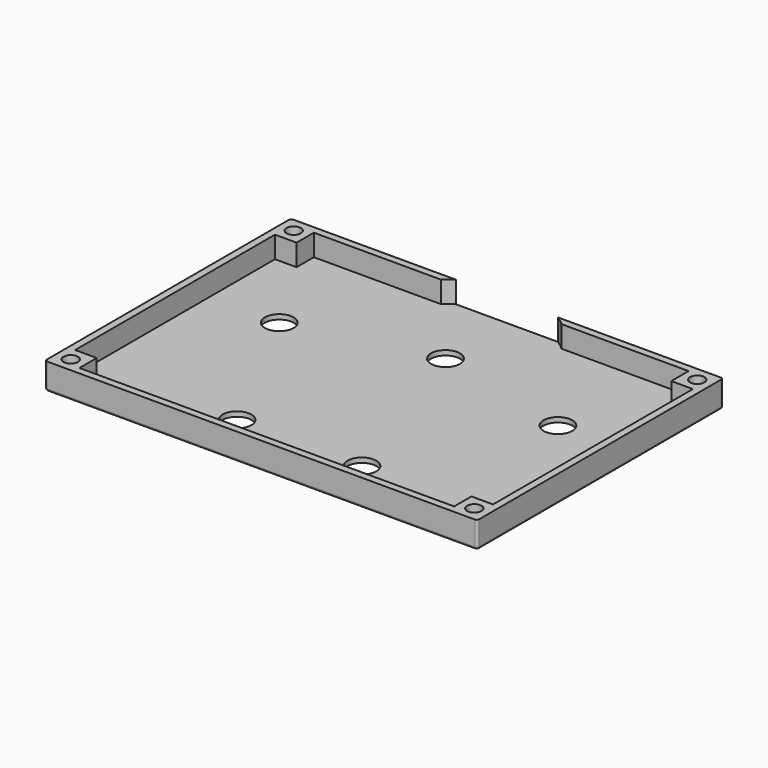
from build123d import *

# Parameters (mm, degrees)
F0_W      = 90
F0_H      = 64
F1_DEPTH  = 1
F3_W      = 90
F3_H      = 64
F3_W_2    = 87
F3_H_2    = 61
F4_DEPTH  = 4.5
F5_R      = 3
F6_DEPTH  = 1.001
F8_DEPTH  = 4.501
F10_W     = 4.5
F10_H     = 4.5
F11_DEPTH = 4.5
F12_R     = 1.5
F13_DEPTH = 5.501
F14_R     = 0.5
F16_SIZE  = 0.2


# Not quite as in the source:
# - two fillets or chamfers of one size are made in one step


with BuildPart() as f1:
    # F0 (on Top) → F1 (new body)
    with BuildSketch(Plane.XY):
        with Locations((45, 32)):
            Rectangle(F0_W, F0_H)
    extrude(amount=F1_DEPTH)

    # F3 (on face) → F4 (join)
    with BuildSketch(Plane.XY.offset(1)):
        with Locations((45, 32)):
            Rectangle(F3_W, F3_H)
        with Locations((45, 32)):
            Rectangle(F3_W_2, F3_H_2, mode=Mode.SUBTRACT)
    extrude(amount=F4_DEPTH)

    # F5 (on face) → F6 (cut, through all)
    with BuildSketch(Plane.XY.offset(1)):
        with Locations((16, 41)):
            Circle(F5_R)
        with Locations((45, 48)):
            Circle(F5_R)
        with Locations((32, 10)):
            Circle(F5_R)
        with Locations((58, 10)):
            Circle(F5_R)
        with Locations((74, 41)):
            Circle(F5_R)
    extrude(amount=-F6_DEPTH, mode=Mode.SUBTRACT)

    # F7 (on face) → F8 (cut, through all)
    with BuildSketch(Plane.XY.offset(1)):
        with BuildLine():
            ThreePointArc((34.3868006709, 64), (35.920722141, 31.0823549641), (64.2, 48))
            ThreePointArc((64.2, 48), (61.9176450359, 57.079277859), (55.6131993291, 64))
            Line((55.6131993291, 64), (34.3868006709, 64))
        make_face()
    extrude(amount=F8_DEPTH, mode=Mode.SUBTRACT)

    # F10 (on face) → F11 (join, through all)
    with BuildSketch(Plane.XY.offset(1)):
        with Locations((86.25, 3.75)):
            Rectangle(F10_W, F10_H)
        with Locations((86.25, 60.25)):
            Rectangle(F10_W, F10_H)
        with Locations((3.75, 3.75)):
            Rectangle(F10_W, F10_H)
        with Locations((3.75, 60.25)):
            Rectangle(F10_W, F10_H)
    extrude(amount=F11_DEPTH)

    # F12 (on face) → F13 (cut, through all)
    with BuildSketch(Plane.XY.offset(5.5)):
        with Locations((87, 3)):
            Circle(F12_R)
        with Locations((3, 3)):
            Circle(F12_R)
        with Locations((87, 61)):
            Circle(F12_R)
        with Locations((3, 61)):
            Circle(F12_R)
    extrude(amount=-F13_DEPTH, mode=Mode.SUBTRACT)

    # F14
    f14_edges = [f1.edges().sort_by_distance(p)[0] for p in [
        (45, 64, 0),
        (0, 64, 2.75),
        (0, 0, 2.75),
        (0, 32, 0),
        (90, 64, 2.75),
        (90, 0, 2.75),
        (45, 0, 0),
        (90, 32, 0),
    ]]
    fillet(f14_edges, radius=F14_R)

    # F16
    f16_edges = [f1.edges().sort_by_distance(p)[0] for p in [
        (85.5, 61, 0),
        (85.5, 3, 0),
        (1.5, 3, 0),
        (1.5, 61, 0),
    ]]
    chamfer(f16_edges, length=F16_SIZE)


solid = f1.part
